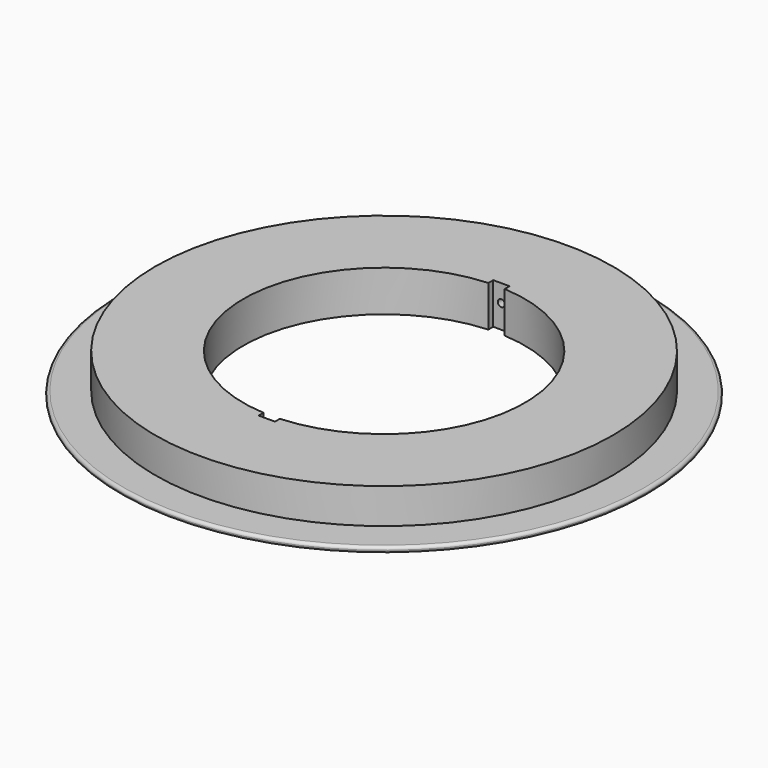
from build123d import *

# Parameters (mm, degrees)
F0_R      = 225
F0_R_2    = 120
F1_DEPTH  = 5
F2_R      = 2.49999
F3_R      = 195
F3_R_2    = 120
F4_DEPTH  = 30
F5_R      = 20
F6_DEPTH  = 15
F8_DEPTH  = 35.001
F10_D     = 6
F10_DEPTH = 20
F10_TIP   = 1.8025818571
F12_D     = 6
F12_DEPTH = 20
F12_TIP   = 1.8025818571


# Not quite as in the source:
# - a fillet or chamfer is up to 0.001 mm smaller than in the source, because OpenCascade refuses the exact size
# - a feature names something its author has since deleted; it is built from what else it names


with BuildPart() as f1:
    # F0 (on Top) → F1 (new body)
    with BuildSketch(Plane.XY):
        Circle(F0_R)
        Circle(F0_R_2, mode=Mode.SUBTRACT)
    extrude(amount=F1_DEPTH)

    # F2 (radius 2.5 in the source; OpenCascade refuses exactly that, so slightly less here)
    f2_edges = [f1.edges().sort_by_distance(p)[0] for p in [
        (-225, 0, 5),
        (-225, 0, 0),
    ]]
    fillet(f2_edges, radius=F2_R)

    # F3 (on face) → F4 (join)
    with BuildSketch(Plane.XY.offset(5)):
        Circle(F3_R)
        Circle(F3_R_2, mode=Mode.SUBTRACT)
    extrude(amount=F4_DEPTH)

    # F5 (on face) → F6 (cut)
    with BuildSketch(Plane(origin=(0, 0, 0), x_dir=(1, 0, 0), z_dir=(0, 0, -1))):
        with BuildLine():
            ThreePointArc((20, 160), (-14.1421356237, 174.1421356237), (0, 140))
            ThreePointArc((0, 140), (14.1421356237, 145.8578643763), (20, 160))
        make_face()
        with Locations((138.5640646055, -80)):
            Circle(F5_R)
        with Locations((-138.5640646055, -80)):
            Circle(F5_R)
    extrude(amount=-F6_DEPTH, mode=Mode.SUBTRACT)

    # F7 (on face) → F8 (cut, through all)
    with BuildSketch(Plane.XY.offset(35)):
        with BuildLine():
            Line((0, 125), (0, 120))
            ThreePointArc((0, 120), (3.501490936, 119.9489039601), (7, 119.7956593538))
            Line((7, 119.7956593538), (7, 125))
            Line((7, 125), (0, 125))
        make_face()
        with BuildLine():
            ThreePointArc((-7, 119.7956593538), (-3.501490936, 119.9489039601), (0, 120))
            Line((0, 120), (0, 125))
            Line((0, 125), (-7, 125))
            Line((-7, 125), (-7, 119.7956593538))
        make_face()
        with BuildLine():
            Line((7, -125), (7, -119.7956593538))
            ThreePointArc((7, -119.7956593538), (3.501490936, -119.9489039601), (0, -120))
            Line((0, -120), (0, -125))
            Line((0, -125), (7, -125))
        make_face()
        with BuildLine():
            ThreePointArc((0, -120), (-3.501490936, -119.9489039601), (-7, -119.7956593538))
            Line((-7, -119.7956593538), (-7, -125))
            Line((-7, -125), (0, -125))
            Line((0, -125), (0, -120))
        make_face()
    extrude(amount=-F8_DEPTH, mode=Mode.SUBTRACT)

    # F10 (one way)
    with BuildSketch(Plane(origin=(0, -125, 0), x_dir=(-1, 0, 0), z_dir=(0, 1, 0))):
        with Locations((0, 20)):
            Circle(F10_D / 2)
    extrude(amount=-F10_DEPTH, mode=Mode.SUBTRACT)
    with Locations(Plane(origin=(0, -125, 0), x_dir=(-1, 0, 0), z_dir=(0, 1, 0))):
        with Locations((0, 20)):
            with Locations((0, 0, -(F10_DEPTH + F10_TIP / 2))):  # 118° drill point
                Cone(0, F10_D / 2, F10_TIP, mode=Mode.SUBTRACT)

    # F12 (one way)
    with BuildSketch(Plane.XZ.offset(-125)):
        with Locations((0, 20)):
            Circle(F12_D / 2)
    extrude(amount=-F12_DEPTH, mode=Mode.SUBTRACT)
    with Locations(Plane.XZ.offset(-125)):
        with Locations((0, 20)):
            with Locations((0, 0, -(F12_DEPTH + F12_TIP / 2))):  # 118° drill point
                Cone(0, F12_D / 2, F12_TIP, mode=Mode.SUBTRACT)


solid = f1.part
